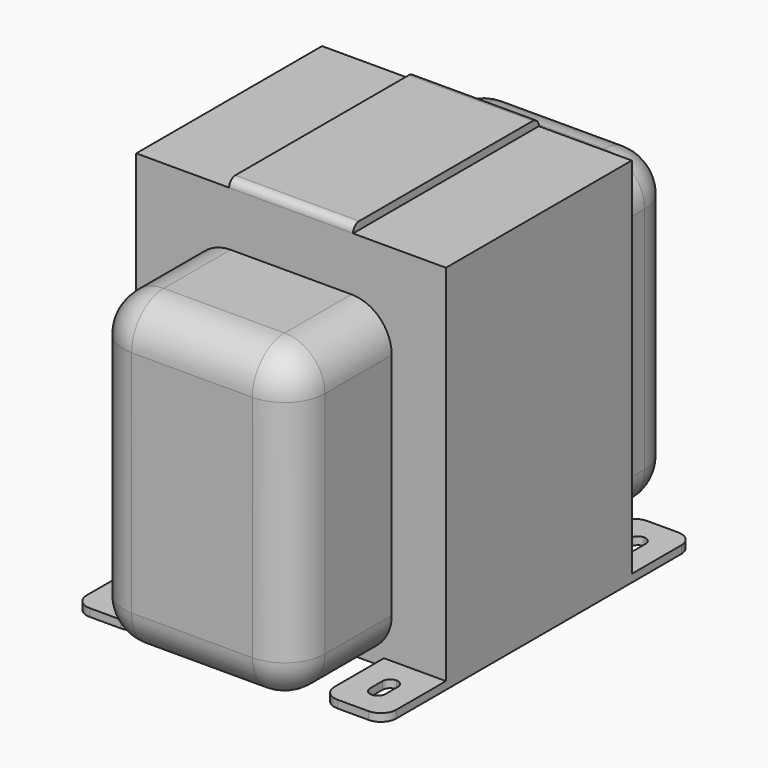
from build123d import *

# Parameters (mm, degrees)
F0_W      = 63.5
F0_H      = 47.625
F1_DEPTH  = 76.2
F2_W      = 41.275
F2_H      = 63.5
F3_DEPTH  = 25.4
F4_R      = 8.255
F6_W      = 12.7
F6_H      = 15.875
F7_DEPTH  = 1.5875
F8_R      = 3.175
F9_W      = 3.175
F9_H      = 6.35
F10_DEPTH = 25.4
F11_R     = 1.58749
F12_W     = 25.4
F12_H     = 47.625
F13_DEPTH = 1.5875
F14_R     = 1.5875


# Not quite as in the source:
# - a fillet or chamfer is up to 0.001 mm smaller than in the source, because OpenCascade refuses the exact size


with BuildPart() as f1:
    # F0 (on Top) → F1 (new body)
    with BuildSketch(Plane.XY):
        Rectangle(F0_W, F0_H)
    extrude(amount=F1_DEPTH)

    # F2 (on face) → F3 (join)
    with BuildSketch(Plane.XZ.offset(23.8125)):
        with Locations((0, 33.3375)):
            Rectangle(F2_W, F2_H)
    extrude(amount=F3_DEPTH)

    # F4
    f4_edges = [f1.edges().sort_by_distance(p)[0] for p in [
        (-20.6375, -36.5125, 65.0875),
        (20.6375, -36.5125, 65.0875),
        (-20.6375, -36.5125, 1.5875),
        (20.6375, -36.5125, 1.5875),
        (20.6375, -49.2125, 33.3375),
        (0, -49.2125, 65.0875),
        (-20.6375, -49.2125, 33.3375),
        (0, -49.2125, 1.5875),
    ]]
    fillet(f4_edges, radius=F4_R)

    # F5: F1 across plane


with BuildPart() as f1_1:
    add(f1.part)
    add(f1.part.mirror(Plane.XZ))

    # F6 (on face) → F7 (join)
    with BuildSketch(Plane(origin=(0, 0, 0), x_dir=(1, 0, 0), z_dir=(0, 0, -1))):
        with Locations((-25.4, 31.75)):
            Rectangle(F6_W, F6_H)
        with Locations((25.4, 31.75)):
            Rectangle(F6_W, F6_H)
        with Locations((25.4, -31.75)):
            Rectangle(F6_W, F6_H)
        with Locations((-25.4, -31.75)):
            Rectangle(F6_W, F6_H)
    extrude(amount=-F7_DEPTH)

    # F8
    f8_edges = [f1_1.edges().sort_by_distance(p)[0] for p in [
        (-31.75, -39.6875, 0.79375),
        (-19.05, -39.6875, 0.79375),
        (19.05, -39.6875, 0.79375),
        (31.75, -39.6875, 0.79375),
        (31.75, 39.6875, 0.79375),
        (19.05, 39.6875, 0.79375),
        (-19.05, 39.6875, 0.79375),
        (-31.75, 39.6875, 0.79375),
    ]]
    fillet(f8_edges, radius=F8_R)

    # F9 (on face) → F10 (cut)
    with BuildSketch(Plane(origin=(0, 0, 0), x_dir=(1, 0, 0), z_dir=(0, 0, -1))):
        with Locations((-25.4, 31.75)):
            Rectangle(F9_W, F9_H)
        with Locations((25.4, 31.75)):
            Rectangle(F9_W, F9_H)
        with Locations((25.4, -31.75)):
            Rectangle(F9_W, F9_H)
        with Locations((-25.4, -31.75)):
            Rectangle(F9_W, F9_H)
    extrude(amount=-F10_DEPTH, mode=Mode.SUBTRACT)

    # F11 (radius 1.5875 in the source; OpenCascade refuses exactly that, so slightly less here)
    f11_edges = [f1_1.edges().sort_by_distance(p)[0] for p in [
        (-26.9875, -34.925, 0.79375),
        (-23.8125, -34.925, 0.79375),
        (-26.9875, -28.575, 0.79375),
        (-23.8125, -28.575, 0.79375),
        (26.9875, -28.575, 0.79375),
        (26.9875, -34.925, 0.79375),
        (23.8125, -34.925, 0.79375),
        (23.8125, -28.575, 0.79375),
        (-26.9875, 34.925, 0.79375),
        (-23.8125, 34.925, 0.79375),
        (-23.8125, 28.575, 0.79375),
        (-26.9875, 28.575, 0.79375),
        (23.8125, 28.575, 0.79375),
        (26.9875, 34.925, 0.79375),
        (23.8125, 34.925, 0.79375),
        (26.9875, 28.575, 0.79375),
    ]]
    fillet(f11_edges, radius=F11_R)

    # F12 (on face) → F13 (join)
    with BuildSketch(Plane.XY.offset(76.2)):
        Rectangle(F12_W, F12_H)
    extrude(amount=F13_DEPTH)

    # F14
    f14_edges = [f1_1.edges().sort_by_distance(p)[0] for p in [
        (0, -23.8125, 77.7875),
        (0, 23.8125, 77.7875),
    ]]
    fillet(f14_edges, radius=F14_R)


solid = f1_1.part
